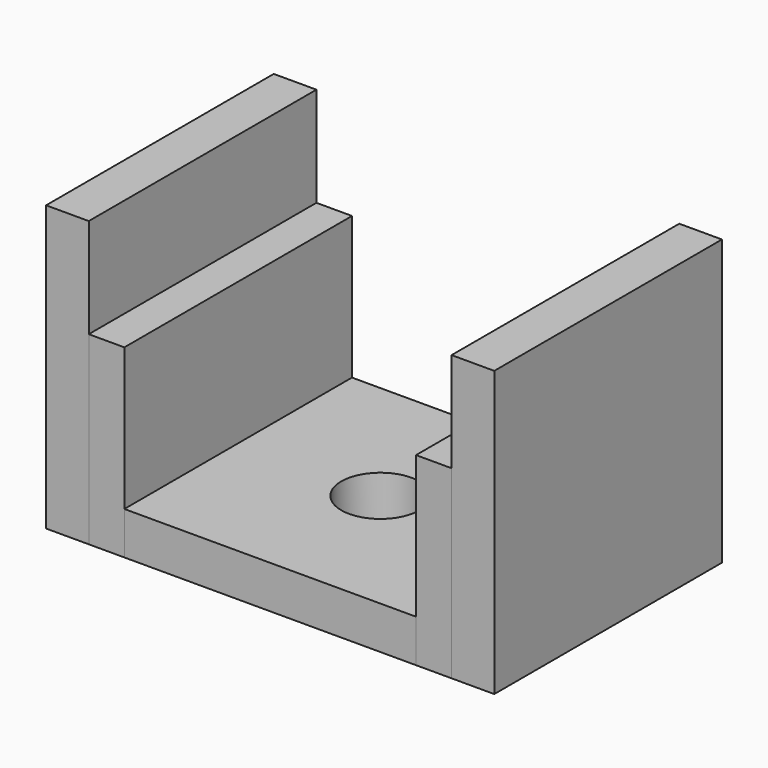
from build123d import *

# Parameters (mm, degrees)
F0_W     = 20.5
F0_H     = 20
F1_DEPTH = 3
F0_W_2   = 3
F2_DEPTH = 20
F3_D     = 5.5
F0_W_3   = 2.5
F4_DEPTH = 13


# Not quite as in the source:
# - a feature names something its author has since deleted; it is built from what else it names


with BuildPart() as f1:
    # F0 (on Top) → F1 (new body)
    with BuildSketch(Plane.XY):
        with Locations((0.2499998137, -1.5457747273)):
            Rectangle(F0_W, F0_H)
    extrude(amount=F1_DEPTH)

    # F3 (through all)
    with Locations(Plane(origin=(0, 0, 0), x_dir=(1, 0, 0), z_dir=(0, 0, -1))):
        with Locations((0, 1.5457747273)):
            Hole(F3_D / 2)


with BuildPart() as f2:
    # F0 (on Top) → F2 (new body)
    with BuildSketch(Plane.XY):
        with Locations((14.4999998137, -1.5457747273)):
            Rectangle(F0_W_2, F0_H)
    extrude(amount=F2_DEPTH)


with BuildPart() as f2b:
    # F0 (on Top) → F2, piece 2 (new body)
    with BuildSketch(Plane.XY):
        with Locations((-14.0000001863, -1.5457747273)):
            Rectangle(F0_W_2, F0_H)
    extrude(amount=F2_DEPTH)


with BuildPart() as f4:
    # F0 (on Top) → F4 (new body)
    with BuildSketch(Plane.XY):
        with Locations((11.7499998137, -1.5457747273)):
            Rectangle(F0_W_3, F0_H)
    extrude(amount=F4_DEPTH)


with BuildPart() as f4b:
    # F0 (on Top) → F4, piece 2 (new body)
    with BuildSketch(Plane.XY):
        with Locations((-11.2500001863, -1.5457747273)):
            Rectangle(F0_W_3, F0_H)
    extrude(amount=F4_DEPTH)


solid = Compound([f1.part, f2.part, f2b.part, f4.part, f4b.part])
